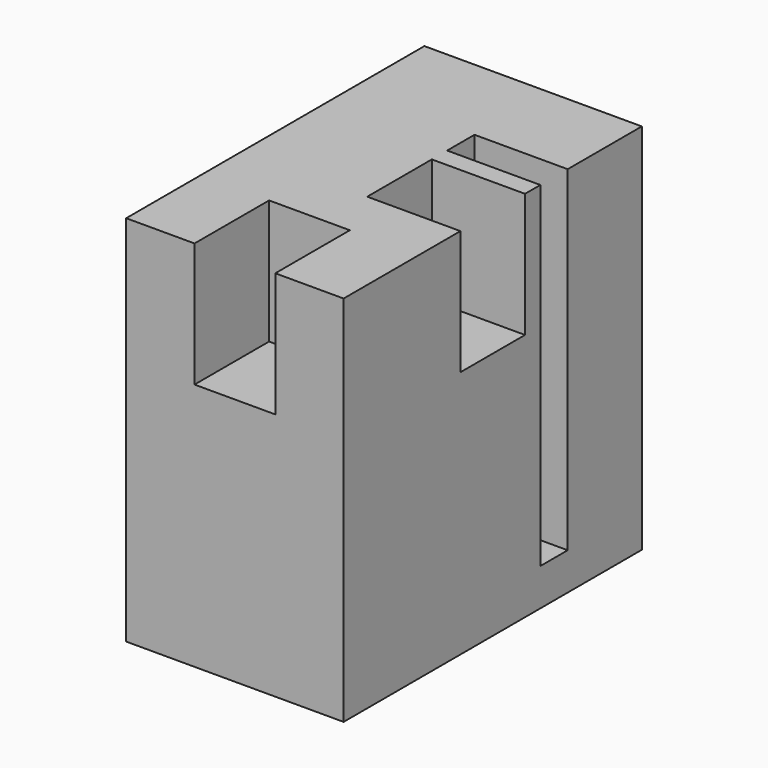
from build123d import *

# Parameters (mm, degrees)
F4_W      = 350
F4_H      = 600
F5_DEPTH  = 600
F6_W      = 130
F6_H      = 150
F6_W_2    = 150
F6_H_2    = 130
F7_DEPTH  = 200
F8_W      = 55
F8_H      = 540
F10_DEPTH = 150


# Not quite as in the source:
# - a feature names something its author has since deleted; it is built from what else it names


with BuildPart() as f5:
    # F4 (on Top) → F5 (new body)
    with BuildSketch(Plane.XY):
        Rectangle(F4_W, F4_H)
    extrude(amount=-F5_DEPTH)

    # F6 (on face) → F7 (cut)
    with BuildSketch(Plane.XY):
        with Locations((0, -225)):
            Rectangle(F6_W, F6_H)
        with Locations((100, 0)):
            Rectangle(F6_W_2, F6_H_2)
    extrude(amount=-F7_DEPTH, mode=Mode.SUBTRACT)

    # F8 (on face) → F10 (cut)
    with BuildSketch(Plane.YZ.offset(175)):
        with Locations((123.3525127172, -270)):
            Rectangle(F8_W, F8_H)
    extrude(amount=-F10_DEPTH, mode=Mode.SUBTRACT)


solid = f5.part
